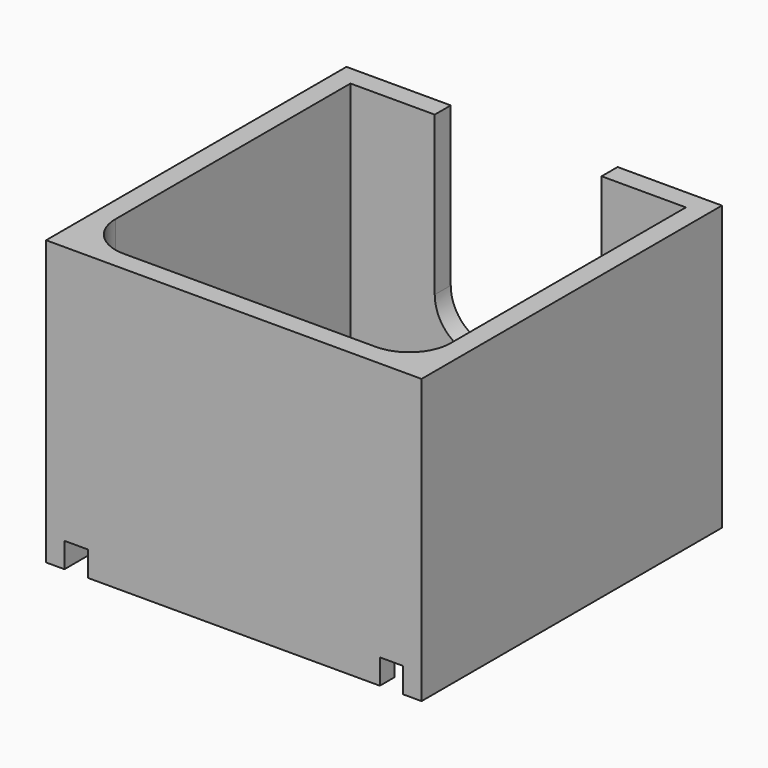
from build123d import *

# Parameters (mm, degrees)
F0_W     = 45
F0_H     = 45
F1_DEPTH = 34
F2_T     = -2.4
F3_R     = 20
F4_R     = 5
F5_W     = 20
F5_H     = 24
F6_DEPTH = 5
F7_R     = 5
F9_DEPTH = 3


with BuildPart() as f1:
    # F0 (on Top) → F1 (new body)
    with BuildSketch(Plane.XY):
        Rectangle(F0_W, F0_H)
    extrude(amount=F1_DEPTH)

    # F2
    f2_openings = [f1.faces().sort_by_distance(p)[0] for p in [
        (0, 0, 34),
    ]]
    offset(amount=F2_T, openings=f2_openings)

    # F3
    f3_edges = [f1.edges().sort_by_distance(p)[0] for p in [
        (0, -20.1, 2.4),
    ]]
    fillet(f3_edges, radius=F3_R)

    # F4
    f4_edges = [f1.edges().sort_by_distance(p)[0] for p in [
        (-20.1, 10, 2.4),
        (20.1, 10, 2.4),
    ]]
    fillet(f4_edges, radius=F4_R)

    # F5 (on face) → F6 (cut)
    with BuildSketch(Plane(origin=(0, 22.5, 0), x_dir=(-1, 0, 0), z_dir=(0, 1, 0))):
        with Locations((0, 22)):
            Rectangle(F5_W, F5_H)
    extrude(amount=-F6_DEPTH, mode=Mode.SUBTRACT)

    # F7
    f7_edges = [f1.edges().sort_by_distance(p)[0] for p in [
        (10, 21.3, 10),
        (-10, 21.3, 10),
    ]]
    fillet(f7_edges, radius=F7_R)

    # F8 (on face) → F9 (cut)
    with BuildSketch(Plane(origin=(0, 0, 0), x_dir=(1, 0, 0), z_dir=(0, 0, -1))):
        Polygon((-17.5, 22.5), (-20.3, 22.5), (-20.3, 20), (-20.3, 17.5), (20.3, 17.5), (20.3, 20), (20.3, 22.5), (17.5, 22.5), (17.5, 20.3), (-17.5, 20.3), align=None)
    extrude(amount=-F9_DEPTH, mode=Mode.SUBTRACT)


solid = f1.part
